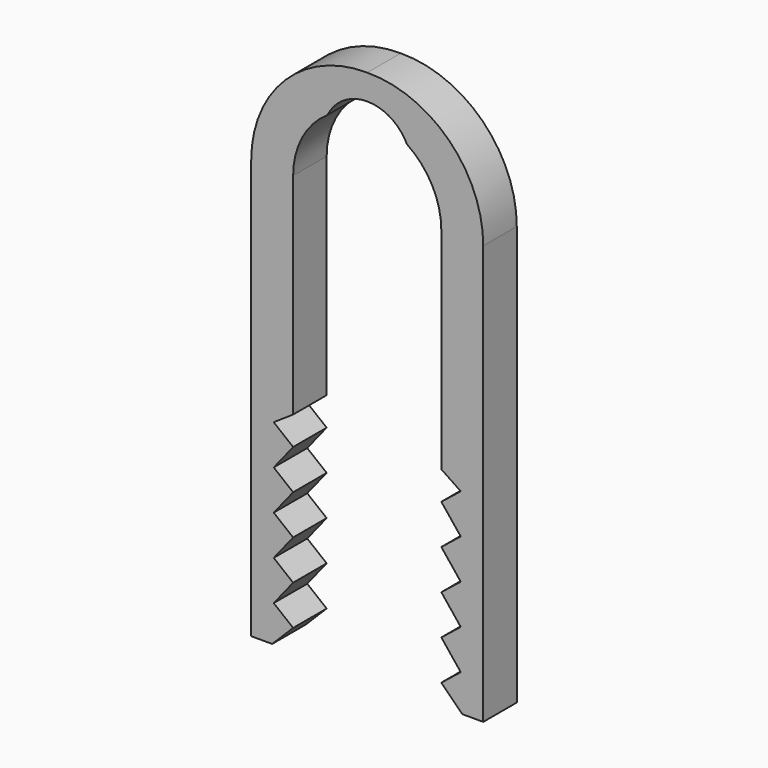
from build123d import *

# Parameters (mm, degrees)
F0_W          = 5.08
F0_H          = 50.8
F1_DEPTH      = 5.08
F4_DEPTH      = 74
F4_DEPTH_BACK = 5.081
F6_DEPTH      = 5.081
F6_DEPTH_BACK = 74


# Not quite as in the source:
# - an extrude ends at something that could not be found from the text; its depth is read off the source's solid
# - a pattern or mirror of a feature is missing from the dataset's text; its kind, count and spacing are read off the source's solid


with BuildPart() as f1:
    # F0 (on Front) → F1 (new body)
    with BuildSketch(Plane.XZ):
        with Locations((-11.5208151574, -9.354611221)):
            Rectangle(F0_W, F0_H)
        with BuildLine():
            ThreePointArc((0, 29.9522848556), (-9.9330623457, 25.933617657), (-14.0608151574, 16.045388779))
            Line((-14.0608151574, 16.045388779), (-8.9808151574, 16.045388779))
            ThreePointArc((-8.9808151574, 16.045388779), (-6.3762662489, 22.555741598), (0, 25.473205834))
            Line((0, 25.473205834), (0, 29.9522848556))
        make_face()
    extrude(amount=F1_DEPTH)

    # F2: F1 across plane


with BuildPart() as f1_1:
    add(f1.part)
    add(f1.part.mirror(Plane.YZ))

    # F3 (on face) → F4 (cut, two sides)
    with BuildSketch(Plane.XZ.offset(5.08)) as f4_sk:
        Polygon((-6.0287490487, -38.7106422752), (-6.0287490487, -7.4653103948), (-11.3340467215, -11.0343284905), (-8.9808151574, -12.9152983427), (-11.3340467215, -15.8593640266), (-8.9808151574, -17.7403338788), (-11.3340467215, -20.6843995627), (-8.9808151574, -22.5653694149), (-11.3340467215, -25.5094350988), (-8.9808151574, -27.390404951), (-11.3340467215, -30.3344706349), (-8.9808151574, -32.2154404871), (-11.5208151574, -34.754611221), (-11.289543082, -38.7106422752), align=None)
    f4 = extrude(amount=F4_DEPTH, mode=Mode.SUBTRACT) + extrude(f4_sk.sketch, amount=-F4_DEPTH_BACK, mode=Mode.SUBTRACT)

    # F4_copies: F4 across plane
    add(f4.mirror(Plane(origin=(0, 0, 0), x_dir=(0, 0, 1), z_dir=(1, 0, 0))), mode=Mode.SUBTRACT)

    # F5 (on face) → F6 (cut, two sides)
    with BuildSketch(Plane.XZ.offset(5.08)) as f6_sk:
        with BuildLine():
            ThreePointArc((0, 25.473205834), (2.5148371028, 25.0039100416), (4.8112860837, 23.8765386418))
            ThreePointArc((4.8112860837, 23.8765386418), (0, 26.8779104299), (-4.8112860837, 23.8765386418))
            ThreePointArc((-4.8112860837, 23.8765386418), (-2.5148371028, 25.0039100416), (0, 25.473205834))
        make_face()
    extrude(amount=-F6_DEPTH, mode=Mode.SUBTRACT)
    extrude(f6_sk.sketch, amount=F6_DEPTH_BACK, mode=Mode.SUBTRACT)


solid = f1_1.part
